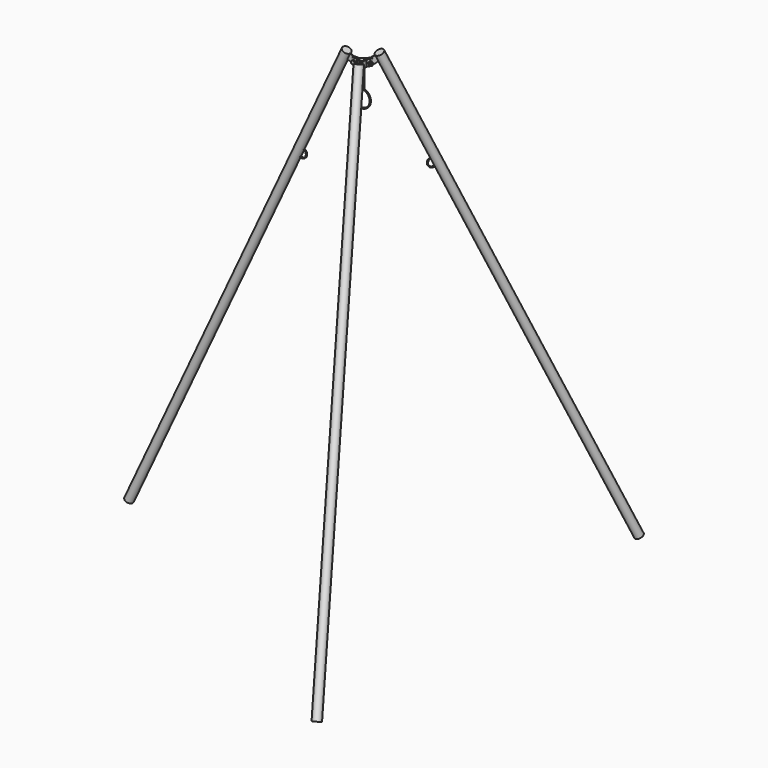
from build123d import *

# Parameters (mm, degrees)
F4_R      = 16
F5_DEPTH  = 2000
F6_R      = 4
F7_DEPTH  = 1.5
F9_DEPTH  = 1.5
F10_COUNT = 3
F12_DEPTH = 12.5
F13_R     = 4
F14_DEPTH = 25
F15_R     = 4
F16_DEPTH = 25
F17_COUNT = 3
F18_R     = 4
F19_DEPTH = 19
F21_DEPTH = 6
F22_R     = 4
F23_DEPTH = 6
F24_COUNT = 3
F25_R     = 8
F26_DEPTH = 100
F28_DEPTH = 1.5


with BuildPart() as f5:
    # F4 (on face) → F5 (new body)
    with BuildSketch(Plane(origin=(0, 0, 0), x_dir=(0.906307787, 0, -0.4226182617), z_dir=(-0.4226182617, 0, -0.906307787))):
        with Locations((-64, 0)):
            Circle(F4_R)
    extrude(amount=F5_DEPTH)


with BuildPart() as f7:
    # F6 (on Front) → F7 (new body, symmetric)
    with BuildSketch(Plane.XZ):
        with BuildLine():
            Line((-54.0682303213, -2.3720181124), (-31.4105356454, -12.9374746559))
            ThreePointArc((-31.4105356454, -12.9374746559), (-14.7989600356, -6.8913555897), (-20.8450791018, 9.72022002))
            Line((-20.8450791018, 9.72022002), (-43.5027737778, 20.2856765636))
            Line((-43.5027737778, 20.2856765636), (-54.0682303213, -2.3720181124))
        make_face()
        with Locations((-26.1278073736, -1.6086273179)):
            Circle(F6_R, mode=Mode.SUBTRACT)
    extrude(amount=F7_DEPTH, both=True)


with BuildPart() as f9:
    # F8 (on Front) → F9 (new body, symmetric)
    with BuildSketch(Plane.XZ):
        with BuildLine():
            Line((-223.1155350176, -364.895132927), (-224.3833898028, -367.6140562881))
            ThreePointArc((-224.3833898028, -367.6140562881), (-217.1280469233, -387.5479470198), (-237.061937655, -394.8032898992))
            Line((-237.061937655, -394.8032898992), (-238.3297924402, -397.5222132603))
            ThreePointArc((-238.3297924402, -397.5222132603), (-214.4091235622, -388.815801805), (-223.1155350176, -364.895132927))
        make_face()
    extrude(amount=F9_DEPTH, both=True)


with BuildPart() as f10_1:
    # F10: instance of F5
    add(f5.part.rotate(Axis((0, 0, 59.7195103765), (0, 0, 1)), 1 * 360 / F10_COUNT))


with BuildPart() as f10_2:
    # F10: instance of F5
    add(f5.part.rotate(Axis((0, 0, 59.7195103765), (0, 0, 1)), 2 * 360 / F10_COUNT))


with BuildPart() as f10_3:
    # F10: instance of F7
    add(f7.part.rotate(Axis((0, 0, 59.7195103765), (0, 0, 1)), 1 * 360 / F10_COUNT))


with BuildPart() as f10_4:
    # F10: instance of F7
    add(f7.part.rotate(Axis((0, 0, 59.7195103765), (0, 0, 1)), 2 * 360 / F10_COUNT))


with BuildPart() as f10_5:
    # F10: instance of F9
    add(f9.part.rotate(Axis((0, 0, 59.7195103765), (0, 0, 1)), 1 * 360 / F10_COUNT))


with BuildPart() as f10_6:
    # F10: instance of F9
    add(f9.part.rotate(Axis((0, 0, 59.7195103765), (0, 0, 1)), 2 * 360 / F10_COUNT))


with BuildPart() as f12:
    # F11 (on Top) → F12 (new body, symmetric)
    with BuildSketch(Plane.XY):
        Polygon((-33.6278073736, 4.5), (-33.6278073736, 1.5), (-13.6278073736, 1.5), (5.5148655811, 12.5520273834), (15.5148655811, 29.8725354591), (12.9167893698, 31.3725354591), (3.3187131584, 14.7481798061), (-14.4316549509, 4.5), align=None)
    extrude(amount=F12_DEPTH, both=True)

    # F13 (on face) → F14 (cut)
    with BuildSketch(Plane.XZ.offset(-1.5)):
        with Locations((-26.1278073736, -1.6086273179)):
            Circle(F13_R)
    extrude(amount=-F14_DEPTH, mode=Mode.SUBTRACT)

    # F15 (on face) → F16 (cut)
    with BuildSketch(Plane(origin=(-1.2990381057, 0.75, 0), x_dir=(0.5, 0.8660254038, 0), z_dir=(0.8660254038, -0.5, 0))):
        with Locations((26.1278073736, -1.6086273179)):
            Circle(F15_R)
    extrude(amount=-F16_DEPTH, mode=Mode.SUBTRACT)


with BuildPart() as f17_1:
    # F17: instance of F12
    add(f12.part.rotate(Axis((0, 0, 59.7195103765), (0, 0, 1)), 1 * 360 / F17_COUNT))


with BuildPart() as f17_2:
    # F17: instance of F12
    add(f12.part.rotate(Axis((0, 0, 59.7195103765), (0, 0, 1)), 2 * 360 / F17_COUNT))


with BuildPart() as f19:
    # F18 (on face) → F19 (new body)
    with BuildSketch(Plane.XZ.offset(4.5)):
        with Locations((-26.1278073736, -1.6086273179)):
            Circle(F18_R)
    extrude(amount=-F19_DEPTH)

    # F20 (on face) → F21 (join)
    with BuildSketch(Plane.XZ.offset(4.5)):
        Polygon((-24.8593749509, -9.0062223678), (-19.0870859221, -4.2089301418), (-20.3555183448, 3.1886649081), (-27.3962397963, 5.788967732), (-33.1685288251, 0.991675506), (-31.9000964024, -6.4059195439), align=None)
    extrude(amount=F21_DEPTH)


with BuildPart() as f23:
    # F22 (on face) → F23 (new body)
    with BuildSketch(Plane(origin=(0, 4.5, 0), x_dir=(-1, 0, 0), z_dir=(0, 1, 0))):
        Polygon((29.8805841233, 4.8913726821), (22.3750306239, 4.8913726821), (18.6222538741, -1.6086273179), (22.3750306239, -8.1086273179), (29.8805841233, -8.1086273179), (33.6333608731, -1.6086273179), align=None)
        with Locations((26.1278073736, -1.6086273179)):
            Circle(F22_R, mode=Mode.SUBTRACT)
    extrude(amount=F23_DEPTH)


with BuildPart() as f24_1:
    # F24: instance of F19
    add(f19.part.rotate(Axis((0, 0, 59.7195103765), (0, 0, 1)), 1 * 360 / F24_COUNT))


with BuildPart() as f24_2:
    # F24: instance of F19
    add(f19.part.rotate(Axis((0, 0, 59.7195103765), (0, 0, 1)), 2 * 360 / F24_COUNT))


with BuildPart() as f24_3:
    # F24: instance of F23
    add(f23.part.rotate(Axis((0, 0, 59.7195103765), (0, 0, 1)), 1 * 360 / F24_COUNT))


with BuildPart() as f24_4:
    # F24: instance of F23
    add(f23.part.rotate(Axis((0, 0, 59.7195103765), (0, 0, 1)), 2 * 360 / F24_COUNT))


with BuildPart() as f26:
    # F25 (on face) → F26 (new body)
    with BuildSketch(Plane.XY.offset(12.5)):
        Circle(F25_R)
    extrude(amount=-F26_DEPTH)


with BuildPart() as f28:
    # F27 (on Front) → F28 (new body, symmetric)
    with BuildSketch(Plane.XZ):
        with BuildLine():
            ThreePointArc((8, -87.5), (0, -150.4838667697), (-8, -87.5))
            Line((-8, -87.5), (-8, -84.4104166949))
            ThreePointArc((-8, -84.4104166949), (0, -153.4838667697), (8, -84.4104166949))
            Line((8, -84.4104166949), (8, -87.5))
        make_face()
    extrude(amount=F28_DEPTH, both=True)


solid = Compound([f5.part, f7.part, f9.part, f10_1.part, f10_2.part, f10_3.part, f10_4.part, f10_5.part, f10_6.part, f12.part, f17_1.part, f17_2.part, f19.part, f23.part, f24_1.part, f24_2.part, f24_3.part, f24_4.part, f26.part, f28.part])
